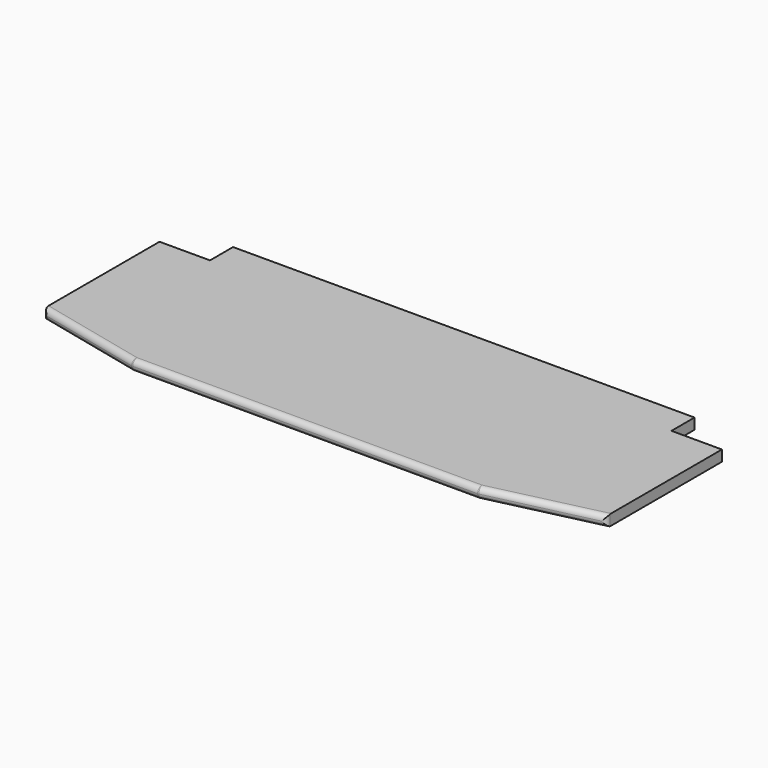
from build123d import *

# Parameters (mm, degrees)
F2_DEPTH = 30
F3_R     = 14.99999


# Not quite as in the source:
# - a fillet or chamfer is up to 0.001 mm smaller than in the source, because OpenCascade refuses the exact size


with BuildPart() as f2:
    # F1 (on offset) → F2 (new body)
    with BuildSketch(Plane.XY.offset(750)):
        Polygon((640, 0), (-640, 0), (-640, -80), (-780, -80), (-780, -480), (-480, -550), (480, -550), (780, -480), (780, -80), (640, -80), align=None)
    extrude(amount=F2_DEPTH)

    # F3 (radius 15 in the source; OpenCascade refuses exactly that, so slightly less here)
    f3_edges = [f2.edges().sort_by_distance(p)[0] for p in [
        (-630, -515, 780),
        (-780, -480, 765),
        (-480, -550, 765),
        (-630, -515, 750),
        (480, -550, 765),
        (0, -550, 750),
        (0, -550, 780),
        (780, -480, 765),
        (630, -515, 750),
        (630, -515, 780),
    ]]
    fillet(f3_edges, radius=F3_R)


solid = f2.part
